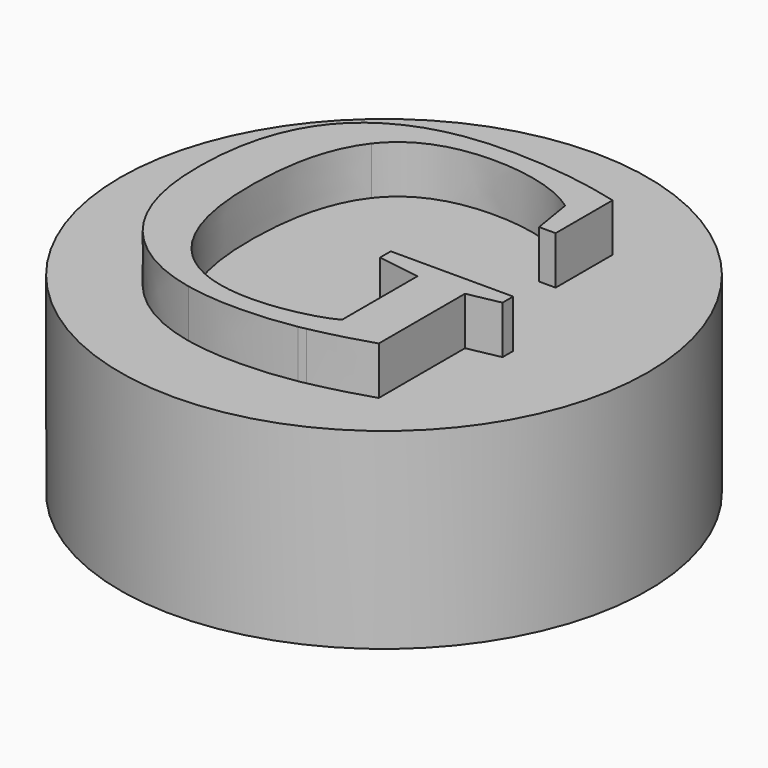
from build123d import *

# Parameters (mm, degrees)
F3_DEPTH = 1.27


with BuildPart() as f1:
    # F0 (on Front) → F1 (revolve)
    with BuildSketch(Plane.XZ):
        with BuildLine():
            Line((-6.985, 6.35), (-6.985, 0))
            Line((-6.985, 0), (-3.81, 0))
            ThreePointArc((-3.81, 0), (-2.6940768363, 2.6940768363), (0, 3.81))
            Line((0, 3.81), (0, 6.35))
            Line((0, 6.35), (-6.985, 6.35))
        make_face()
    revolve(axis=Axis((0, 0, 5.08), (0, 0, 1)))

    # F2 (on face) → F3 (cut)
    with BuildSketch(Plane.XY.offset(6.35)):
        with BuildLine():
            Line((-5.0499272347, 4.825811841), (5.0499272347, 4.825811841))
            ThreePointArc((5.0499272347, 4.825811841), (0, 6.985), (-5.0499272347, 4.825811841))
        make_face()
        with BuildLine():
            Line((5.0499272347, -4.825811841), (5.0499272347, 4.825811841))
            Line((5.0499272347, 4.825811841), (-5.0499272347, 4.825811841))
            Line((-5.0499272347, 4.825811841), (-5.0499272347, -4.825811841))
            Line((-5.0499272347, -4.825811841), (-1.3193129815, -4.825811841))
            add(Edge.make_bspline(
                [(-1.3193129815, -4.825811841), (-2.5203953314, -4.5677027566), (-3.3083202269, -3.8047253512)],
                knots=[0.3382919108, 0.3382919108, 0.3382919108, 1, 1, 1], degree=2))
            add(Edge.make_bspline(
                [(-3.3083202269, -3.8047253512), (-4.4990641643, -2.6516830689), (-4.4990641643, -0.5382958521)],
                knots=[0, 0, 0, 1, 1, 1], degree=2))
            add(Edge.make_bspline(
                [(-4.4990641643, -0.5382958521), (-4.4990641643, 1.7656941762), (-3.3439273456, 2.9082637766)],
                knots=[0, 0, 0, 1, 1, 1], degree=2))
            add(Edge.make_bspline(
                [(-3.3439273456, 2.9082637766), (-2.1887905268, 4.0508333769), (0.0418907278, 4.0508333769)],
                knots=[0, 0, 0, 1, 1, 1], degree=2))
            add(Edge.make_bspline(
                [(0.0418907278, 4.0508333769), (1.6400219928, 4.0508333769), (3.1250482929, 3.6570605358)],
                knots=[0, 0, 0, 1, 1, 1], degree=2))
            Line((3.1250482929, 3.6570605358), (3.1250482929, 1.7719777854))
            Line((3.1250482929, 1.7719777854), (2.6872901875, 1.7719777854))
            Line((2.6872901875, 1.7719777854), (2.5092545944, 2.8590421714))
            add(Edge.make_bspline(
                [(2.5092545944, 2.8590421714), (2.0589292707, 3.179506239), (1.4274265493, 3.3533527593)],
                knots=[0, 0, 0, 1, 1, 1], degree=2))
            add(Edge.make_bspline(
                [(1.4274265493, 3.3533527593), (0.7959238279, 3.5271992796), (0.0942541375, 3.5271992796)],
                knots=[0, 0, 0, 1, 1, 1], degree=2))
            add(Edge.make_bspline(
                [(0.0942541375, 3.5271992796), (-1.5813749739, 3.5271992796), (-2.356353438, 2.5281054219)],
                knots=[0, 0, 0, 1, 1, 1], degree=2))
            add(Edge.make_bspline(
                [(-2.356353438, 2.5281054219), (-3.131331902, 1.5290115642), (-3.131331902, -0.5257286337)],
                knots=[0, 0, 0, 1, 1, 1], degree=2))
            add(Edge.make_bspline(
                [(-3.131331902, -0.5257286337), (-3.131331902, -2.4568911847), (-2.3333135377, -3.4549377742)],
                knots=[0, 0, 0, 1, 1, 1], degree=2))
            add(Edge.make_bspline(
                [(-2.3333135377, -3.4549377742), (-1.5352951734, -4.4529843637), (0.0293235095, -4.4529843637)],
                knots=[0, 0, 0, 1, 1, 1], degree=2))
            add(Edge.make_bspline(
                [(0.0293235095, -4.4529843637), (0.5801865798, -4.4529843637), (1.1823657918, -4.3220758394)],
                knots=[0, 0, 0, 1, 1, 1], degree=2))
            add(Edge.make_bspline(
                [(1.1823657918, -4.3220758394), (1.7845450037, -4.191167315), (2.0987254621, -4.0068481128)],
                knots=[0, 0, 0, 1, 1, 1], degree=2))
            Line((2.0987254621, -4.0068481128), (2.0987254621, -1.5143498095))
            Line((2.0987254621, -1.5143498095), (0.9718648846, -1.3425978256))
            Line((0.9718648846, -1.3425978256), (0.9718648846, -0.9907157121))
            Line((0.9718648846, -0.9907157121), (4.2121126789, -0.9907157121))
            Line((4.2121126789, -0.9907157121), (4.2121126789, -1.3425978256))
            Line((4.2121126789, -1.3425978256), (3.3554472957, -1.5143498095))
            Line((3.3554472957, -1.5143498095), (3.3554472957, -4.3671083717))
            add(Edge.make_bspline(
                [(3.3554472957, -4.3671083717), (2.5951305864, -4.6163582021), (1.7772141263, -4.7870629178)],
                knots=[0, 0, 0, 1, 1, 1], degree=2))
            add(Edge.make_bspline(
                [(1.7772141263, -4.7870629178), (1.6784160951, -4.8076827374), (1.5777996884, -4.825811841)],
                knots=[0, 0, 0, 0.1207923255, 0.1207923255, 0.1207923255], degree=2))
            Line((1.5777996884, -4.825811841), (5.0499272347, -4.825811841))
        make_face()
        with BuildLine():
            Line((-5.0499272347, -4.825811841), (-5.0499272347, 4.825811841))
            ThreePointArc((-5.0499272347, 4.825811841), (-6.985, 0), (-5.0499272347, -4.825811841))
        make_face()
        with BuildLine():
            ThreePointArc((-5.0499272347, -4.825811841), (0, -6.985), (5.0499272347, -4.825811841))
            Line((5.0499272347, -4.825811841), (1.5777996884, -4.825811841))
            add(Edge.make_bspline(
                [(1.5777996884, -4.825811841), (0.8454459018, -4.9577676335), (0.0167562911, -4.9577676335)],
                knots=[0.1207923255, 0.1207923255, 0.1207923255, 1, 1, 1], degree=2))
            add(Edge.make_bspline(
                [(0.0167562911, -4.9577676335), (-0.7052711558, -4.9577676335), (-1.3193129815, -4.825811841)],
                knots=[0, 0, 0, 0.3382919108, 0.3382919108, 0.3382919108], degree=2))
            Line((-1.3193129815, -4.825811841), (-5.0499272347, -4.825811841))
        make_face()
        with BuildLine():
            ThreePointArc((6.985, 0), (6.4832077992, 2.5996618305), (5.0499272347, 4.825811841))
            Line((5.0499272347, 4.825811841), (5.0499272347, -4.825811841))
            ThreePointArc((5.0499272347, -4.825811841), (6.4832077992, -2.5996618305), (6.985, 0))
        make_face()
    extrude(amount=-F3_DEPTH, mode=Mode.SUBTRACT)


solid = f1.part
